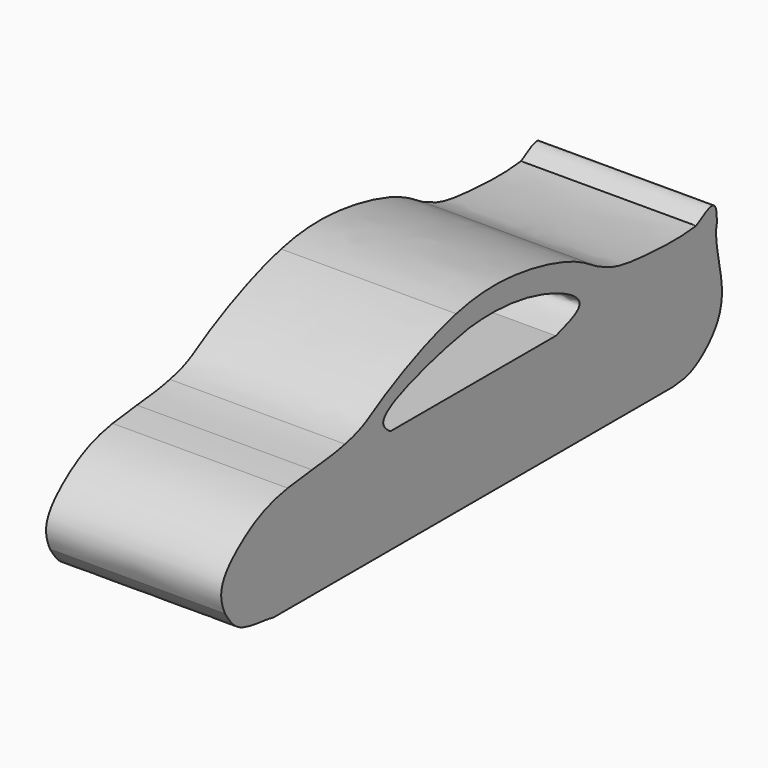
from build123d import *

# Parameters (mm, degrees)
F1_DEPTH = 40


with BuildPart() as f1:
    # F0 (on Right) → F1 (new body)
    with BuildSketch(Plane.YZ):
        with BuildLine():
            add(Edge.make_bspline(
                [(-44.838704501, -6.3841724768), (-46.8453205455, -5.825457283), (-55.6681341229, -5.7726866527), (-57.7306464731, -1.4179735635), (-58.7613759126, 0)],
                knots=[0, 0, 0, 0, 0.5626960778, 1, 1, 1, 1], degree=3))
            Line((-44.838704501, -6.3841724768), (69.161295499, -6.3841724768))
            add(Edge.make_bspline(
                [(69.161295499, -6.3841724768), (71.4475678954, -6.1729190484), (74.6946425338, -5.8699737813), (81.8275271025, -0.1960649024), (84.2715006558, 8.1620243826), (80.7845015237, 18.3321377417), (81.6652249495, 21.4803665876)],
                knots=[0, 0, 0, 0, 0.0810771817, 0.1783295809, 0.2792067504, 0.4028908662, 0.4028908662, 0.4028908662, 0.4028908662], degree=3))
            add(Edge.make_bspline(
                [(81.6374216797, 22.4453190982), (81.6500654198, 22.1293211952), (81.6576451847, 21.8048438914), (81.6652249495, 21.4803665876)],
                knots=[0.9139943138, 0.9139943138, 0.9139943138, 0.9139943138, 1, 1, 1, 1], degree=3))
            add(Edge.make_bspline(
                [(75.7401209274, 23.3199857175), (78.0850621891, 23.5805863979), (81.1237295684, 23.990384777), (81.6374216797, 22.4453190982)],
                knots=[0.7859721691, 0.7859721691, 0.7859721691, 0.7859721691, 0.9689675221, 0.9689675221, 0.9689675221, 0.9689675221], degree=3))
            add(Edge.make_bspline(
                [(47.8096007504, 26.4636462757), (50.4151132719, 25.2566612425), (54.0270677376, 23.6070629686), (68.3082992802, 22.7847875979), (72.6222400219, 22.9734858293), (75.7401209274, 23.3199857175)],
                knots=[0, 0, 0, 0, 0.2310309702, 0.5426578797, 0.7859721691, 0.7859721691, 0.7859721691, 0.7859721691], degree=3))
            add(Edge.make_bspline(
                [(47.8096007504, 26.4636462757), (38.9469496949, 27.2014516696), (19.8383470871, 30.9230949853), (7.2381034379, 33.4919049177)],
                knots=[0.7500808852, 0.7500808852, 0.7500808852, 0.7500808852, 0.9114828872, 0.9114828872, 0.9114828872, 0.9114828872], degree=3))
            add(Edge.make_bspline(
                [(7.2381034379, 33.4919049177), (7.0293313069, 33.4424692791), (-0.6619575082, 31.5703885813), (-15.3393975904, 24.8264789662), (-19.5332629376, 21.2280452336), (-24.5166032072, 20.1923100725)],
                knots=[0.4361701211, 0.4361701211, 0.4361701211, 0.4361701211, 0.4414328852, 0.6293645181, 0.7611494878, 0.7611494878, 0.7611494878, 0.7611494878], degree=3))
            add(Edge.make_bspline(
                [(-24.5166032072, 20.1923100725), (-27.1952683602, 19.5284516677), (-30.5343573496, 19.1890804899), (-33.9337619399, 18.8384775563)],
                knots=[0, 0, 0, 0, 0.1548207433, 0.1548207433, 0.1548207433, 0.1548207433], degree=3))
            add(Edge.make_bspline(
                [(-33.9337619399, 18.8384775563), (-36.1619029939, 18.5738236368), (-38.5117720873, 18.2998204972), (-40.8694513595, 17.9847684884)],
                knots=[0.82699703, 0.82699703, 0.82699703, 0.82699703, 0.867474623, 0.867474623, 0.867474623, 0.867474623], degree=3))
            add(Edge.make_bspline(
                [(-40.8694513595, 17.9847684884), (-41.7301591235, 17.843002501), (-47.4822650158, 16.7449192121), (-54.3846967183, 12.8459477913), (-60.8683867647, 6.2520742648), (-59.4702371494, 1.5500023351), (-58.7613759126, 0)],
                knots=[0.2618071145, 0.2618071145, 0.2618071145, 0.2618071145, 0.3034989867, 0.5490089029, 0.7603362688, 0.8611758874, 0.8611758874, 0.8611758874, 0.8611758874], degree=3))
        make_face()
        with BuildLine():
            add(Edge.make_bspline(
                [(10.9806247056, 29.136126861), (7.2108730674, 28.4910239279), (-0.4322852797, 26.9914683958), (-17.0990938919, 21.1353577397), (-11.5334123789, 17.4561242614), (-11.4637765201, 17.4852853631), (-11.4568779245, 17.4886267632)],
                knots=[0, 0, 0, 0, 0.3909237382, 0.7850289694, 0.9782824352, 1, 1, 1, 1], degree=3))
            add(Edge.make_bspline(
                [(35.6915146112, 17.4886267632), (36.7587346212, 17.9547515009), (47.3920951695, 20.4782306051), (31.2295468414, 28.9607742297), (18.3165498499, 29.9648338159), (10.9806247056, 29.136126861)],
                knots=[0, 0, 0, 0, 0.2520150835, 0.5614741686, 1, 1, 1, 1], degree=3))
            Line((35.6915146112, 17.4886267632), (21.6614138335, 17.4886267632))
            Line((21.6614138335, 17.4886267632), (-11.4568779245, 17.4886267632))
        make_face(mode=Mode.SUBTRACT)
        with BuildLine():
            add(Edge.make_bspline(
                [(-33.9337619399, 18.8384775563), (-36.2828655116, 18.5961990685), (-38.6607714567, 18.3485571057), (-40.8694513595, 17.9847684884)],
                knots=[0.1548207433, 0.1548207433, 0.1548207433, 0.1548207433, 0.2618071145, 0.2618071145, 0.2618071145, 0.2618071145], degree=3))
            add(Edge.make_bspline(
                [(-33.9337619399, 18.8384775563), (-36.1619029939, 18.5738236368), (-38.5117720873, 18.2998204972), (-40.8694513595, 17.9847684884)],
                knots=[0.82699703, 0.82699703, 0.82699703, 0.82699703, 0.867474623, 0.867474623, 0.867474623, 0.867474623], degree=3))
        make_face()
        with BuildLine():
            add(Edge.make_bspline(
                [(47.8096007504, 26.4636462757), (38.9469496949, 27.2014516696), (19.8383470871, 30.9230949853), (7.2381034379, 33.4919049177)],
                knots=[0.7500808852, 0.7500808852, 0.7500808852, 0.7500808852, 0.9114828872, 0.9114828872, 0.9114828872, 0.9114828872], degree=3))
            add(Edge.make_bspline(
                [(47.8096007504, 26.4636462757), (45.3407789538, 28.0318315658), (40.389939725, 31.0970656548), (25.1323891576, 35.0557908721), (13.8550573864, 35.0587488343), (7.2381034379, 33.4919049177)],
                knots=[0, 0, 0, 0, 0.1156638206, 0.269368798, 0.4361701211, 0.4361701211, 0.4361701211, 0.4361701211], degree=3))
        make_face()
        with BuildLine():
            add(Edge.make_bspline(
                [(75.7401209274, 23.3199857175), (78.0850621891, 23.5805863979), (81.1237295684, 23.990384777), (81.6374216797, 22.4453190982)],
                knots=[0.7859721691, 0.7859721691, 0.7859721691, 0.7859721691, 0.9689675221, 0.9689675221, 0.9689675221, 0.9689675221], degree=3))
            add(Edge.make_bspline(
                [(75.7401209274, 23.3199857175), (77.7663103657, 24.605784142), (81.2120858063, 26.792436855), (81.582065434, 23.8288066823), (81.6374216797, 22.4453190982)],
                knots=[0, 0, 0, 0, 0.5374481469, 0.9139943138, 0.9139943138, 0.9139943138, 0.9139943138], degree=3))
        make_face()
    extrude(amount=F1_DEPTH)


solid = f1.part
